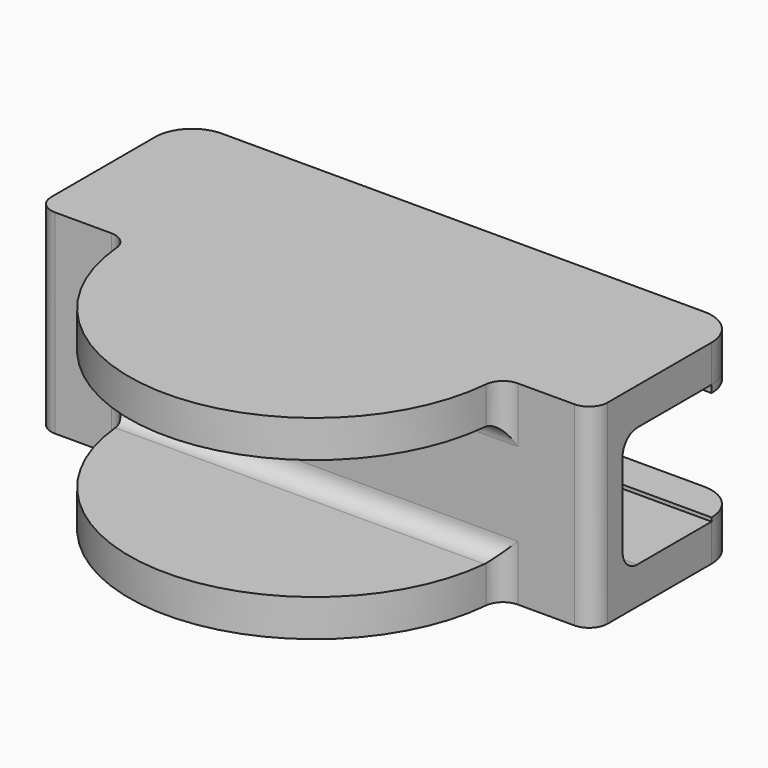
from build123d import *

# Parameters (mm, degrees)
F0_W      = 30
F0_H      = 10
F1_DEPTH  = 2
F2_W      = 30
F2_H      = 2
F3_DEPTH  = 6.5
F4_W      = 30
F4_H      = 10
F5_DEPTH  = 2
F6_R      = 2
F8_DEPTH  = 0.2
F10_DEPTH = 0.4
F12_DEPTH = 2
F14_DEPTH = 2
F15_R     = 1


with BuildPart() as f1:
    # F0 (on Top) → F1 (new body)
    with BuildSketch(Plane.XY):
        with Locations((15, 5)):
            Rectangle(F0_W, F0_H)
    extrude(amount=F1_DEPTH)

    # F2 (on face) → F3 (join)
    with BuildSketch(Plane.XY.offset(2)):
        with Locations((15, 1)):
            Rectangle(F2_W, F2_H)
    extrude(amount=F3_DEPTH)

    # F4 (on face) → F5 (join)
    with BuildSketch(Plane.XY.offset(8.5)):
        with Locations((15, 5)):
            Rectangle(F4_W, F4_H)
    extrude(amount=F5_DEPTH)

    # F6
    f6_edges = [f1.edges().sort_by_distance(p)[0] for p in [
        (30, 10, 9.5),
        (30, 10, 1),
        (0, 10, 9.5),
        (0, 10, 1),
    ]]
    fillet(f6_edges, radius=F6_R)

    # F7 (on face) → F8 (join)
    with BuildSketch(Plane.XY.offset(2)):
        with BuildLine():
            Line((28, 10), (2, 10))
            ThreePointArc((2, 10), (0.5857864376, 9.4142135624), (0, 8))
            Line((0, 8), (30, 8))
            ThreePointArc((30, 8), (29.4142135624, 9.4142135624), (28, 10))
        make_face()
    extrude(amount=F8_DEPTH)

    # F9 (on face) → F10 (join)
    with BuildSketch(Plane(origin=(0, 0, 8.5), x_dir=(1, 0, 0), z_dir=(0, 0, -1))):
        with BuildLine():
            ThreePointArc((0, -8), (0.5857864376, -9.4142135624), (2, -10))
            Line((2, -10), (28, -10))
            ThreePointArc((28, -10), (29.4142135624, -9.4142135624), (30, -8))
            Line((30, -8), (0, -8))
        make_face()
    extrude(amount=F10_DEPTH)

    # F11 (on face) → F12 (join, through all)
    with BuildSketch(Plane.XY.offset(10.5)):
        with BuildLine():
            Line((25, 0), (15, 0))
            Line((15, 0), (5, 0))
            ThreePointArc((5, 0), (15, -10), (25, 0))
        make_face()
    extrude(amount=-F12_DEPTH)

    # F13 (on face) → F14 (join, through all)
    with BuildSketch(Plane(origin=(0, 0, 0), x_dir=(1, 0, 0), z_dir=(0, 0, -1))):
        with BuildLine():
            ThreePointArc((25, 0), (15, 10), (5, 0))
            Line((5, 0), (25, 0))
        make_face()
    extrude(amount=-F14_DEPTH)

    # F15
    f15_edges = [f1.edges().sort_by_distance(p)[0] for p in [
        (15, 0, 2),
        (15, 0, 8.5),
        (5, 0, 9.5),
        (5, 0, 1),
        (25, 0, 9.5),
        (30, 0, 5.25),
        (0, 0, 5.25),
        (15, 2, 2),
        (15, 2, 8.5),
        (25, 0, 1),
    ]]
    fillet(f15_edges, radius=F15_R)


solid = f1.part
